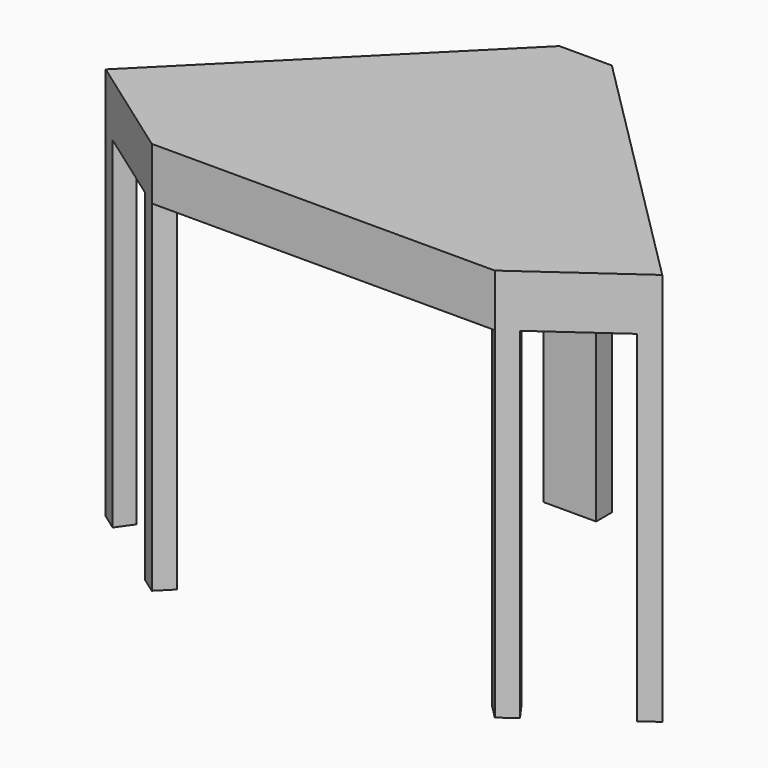
from build123d import *

# Parameters (mm, degrees)
F1_DEPTH = 101.6
F2_W     = 101.6
F2_H     = 38.1
F3_DEPTH = 762
F4_W     = 177.4056817709
F4_H     = 660.4
F5_DEPTH = 76.2


# Not quite as in the source:
# - a pattern or mirror of a feature is missing from the dataset's text; its kind, count and spacing are read off the source's solid


with BuildPart() as f1:
    # F0 (on Top) → F1 (new body)
    with BuildSketch(Plane.XY):
        Polygon((332.1480994978, 125.0519005022), (228.6, 228.6), (0, 228.6), (-228.6, 228.6), (-332.1480994978, 125.0519005022), (-332.1480994978, -228.6), (-228.6, -228.6), (228.6, -228.6), (332.1480994978, -228.6), align=None)
        Polygon((-228.6, 228.6), (0, 228.6), (0, 406.4), (-50.8, 406.4), align=None)
        Polygon((0, 228.6), (228.6, 228.6), (50.8, 406.4), (0, 406.4), align=None)
        Polygon((538.8153672641, -81.6153672641), (332.1480994978, 125.0519005022), (332.1480994978, -228.6), align=None)
        Polygon((-332.1480994978, -228.6), (-332.1480994978, 125.0519005022), (-538.8153672641, -81.6153672641), align=None)
    extrude(amount=F1_DEPTH)

    # F2 (on face) → F3 (join)
    with BuildSketch(Plane.XY.offset(101.6)):
        Polygon((-511.8745989009, -54.6745989009), (-538.8153672641, -81.6153672641), (-332.1480994978, -228.6), (-305.2073311346, -201.6592316368), align=None)
        Polygon((305.2073311346, -201.6592316368), (332.1480994978, -228.6), (538.8153672641, -81.6153672641), (511.8745989009, -54.6745989009), align=None)
        with Locations((0, 387.35)):
            Rectangle(F2_W, F2_H)
    extrude(amount=-F3_DEPTH)

    # F4 (on face) → F5 (cut)
    with BuildSketch(Plane(origin=(219.5423321657, -308.6867865247, 0), x_dir=(0.8149157634, 0.5795794152, 0), z_dir=(0.5795794152, -0.8149157634, 0))):
        with Locations((264.983708636, -330.2)):
            Rectangle(F4_W, F4_H)
    f5 = extrude(amount=-F5_DEPTH, mode=Mode.SUBTRACT)

    # F5_copies: F5 across plane
    add(f5.mirror(Plane(origin=(0, 0, 0), x_dir=(0, 0, -1), z_dir=(-1, 0, 0))), mode=Mode.SUBTRACT)


solid = f1.part
